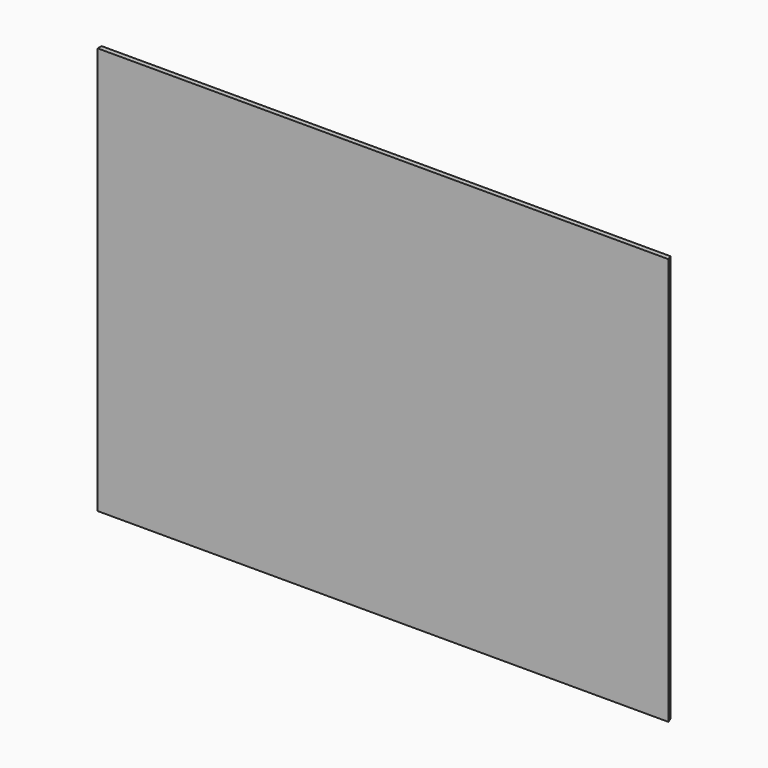
from build123d import *

# Parameters (mm, degrees)
F0_W     = 1476.9619122421
F0_H     = 1054.1
F1_DEPTH = 12.7
F2_SIZE2 = 5.260502
F2_SIZE  = 12.69999


# Not quite as in the source:
# - a fillet or chamfer is up to 0.001 mm smaller than in the source, because OpenCascade refuses the exact size


with BuildPart() as f1:
    # F0 (on Front) → F1 (new body)
    with BuildSketch(Plane.XZ):
        with Locations((738.4809561211, 527.05)):
            Rectangle(F0_W, F0_H)
    extrude(amount=-F1_DEPTH)

    # F2 (size 12.7 and 5.2605122421 in the source; OpenCascade refuses exactly that, so slightly less here)
    f2_edges = [f1.edges().sort_by_distance(p)[0] for p in [
        (1476.961912, 12.7, 527.05),
    ]]
    f2_side = f1.faces().sort_by_distance((1476.961912, 6.35, 527.05))[0]
    chamfer(f2_edges, length=F2_SIZE, length2=F2_SIZE2, reference=f2_side)


solid = f1.part
